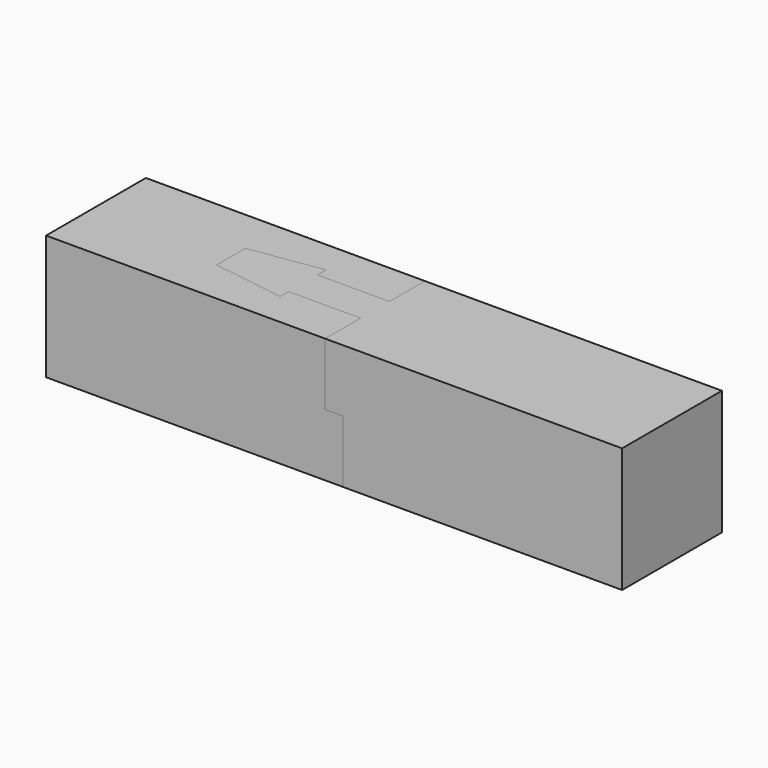
from build123d import *

# Parameters (mm, degrees)
F0_W          = 250
F0_H          = 105
F1_DEPTH      = 52.5
F2_W          = 105
F2_H          = 52.5
F3_DEPTH      = 15.15
F5_DEPTH      = 52.5
F6_W          = 250
F6_H          = 105
F7_DEPTH      = 52.5
F7_DEPTH_BACK = 52.5


with BuildPart() as f1:
    # F0 (on Top) → F1 (new body, symmetric)
    with BuildSketch(Plane.XY):
        with Locations((125, 0)):
            Rectangle(F0_W, F0_H)
    extrude(amount=F1_DEPTH, both=True)

    # F2 (on face) → F3 (cut)
    with BuildSketch(Plane(origin=(0, 0, 0), x_dir=(0, -1, 0), z_dir=(-1, 0, 0))):
        with Locations((0, -26.25)):
            Rectangle(F2_W, F2_H)
    extrude(amount=-F3_DEPTH, mode=Mode.SUBTRACT)

    # F4 (on face) → F5 (join, through all)
    with BuildSketch(Plane.XY.offset(52.5)):
        Polygon((0, -15.15), (0, 15.15), (-60.6, 15.15), (-60.6, 24.24), (-121.2, 15.15), (-121.2, -15.15), (-60.6, -24.24), (-60.6, -15.15), align=None)
    extrude(amount=-F5_DEPTH)


with BuildPart() as f7:
    # F6 (on Top) → F7 (new body, two sides)
    with BuildSketch(Plane.XY) as f7_sk:
        with Locations((-109.85, 0)):
            Rectangle(F6_W, F6_H)
    extrude(amount=F7_DEPTH)
    extrude(f7_sk.sketch, amount=-F7_DEPTH_BACK)

    # F8: cut F1
    add(f1.part, mode=Mode.SUBTRACT)


solid = Compound([f1.part, f7.part])
